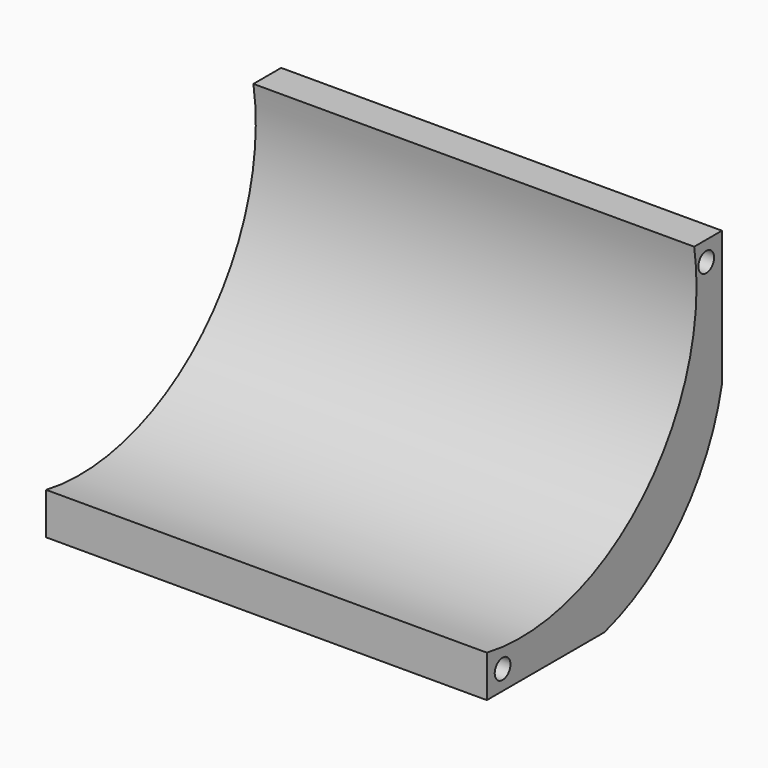
from build123d import *

# Parameters (mm, degrees)
F0_W     = 114.3
F0_H     = 76.2
F1_DEPTH = 76.2
F2_R     = 2.5527
F3_DEPTH = 114.3


# Not quite as in the source:
# - a feature names something its author has since deleted; it is built from what else it names


with BuildPart() as f1:
    # F0 (on Front) → F1 (new body)
    with BuildSketch(Plane.XZ):
        with Locations((0.8173113427, -2.9648756608)):
            Rectangle(F0_W, F0_H)
    extrude(amount=F1_DEPTH)

    # F2 (on face) → F3 (cut)
    with BuildSketch(Plane.YZ.offset(57.9673113427)):
        with Locations((-71.0946, -35.9848756608)):
            Circle(F2_R)
        with Locations((-5.08, 30.0551243392)):
            Circle(F2_R)
        with BuildLine():
            ThreePointArc((0, 0), (-13.3911011826, -25.7827653055), (-38.1, -41.0648756608))
            Line((-38.1, -41.0648756608), (0, -41.0648756608))
            Line((0, -41.0648756608), (0, 0))
        make_face()
        with BuildLine():
            Line((-76.2, 35.1351243392), (-76.2, -30.2226077765))
            ThreePointArc((-76.2, -30.2226077765), (-25.506077145, -15.1181602946), (-8.9947013184, 35.1351243392))
            Line((-8.9947013184, 35.1351243392), (-76.2, 35.1351243392))
        make_face()
    extrude(amount=-F3_DEPTH, mode=Mode.SUBTRACT)


solid = f1.part
